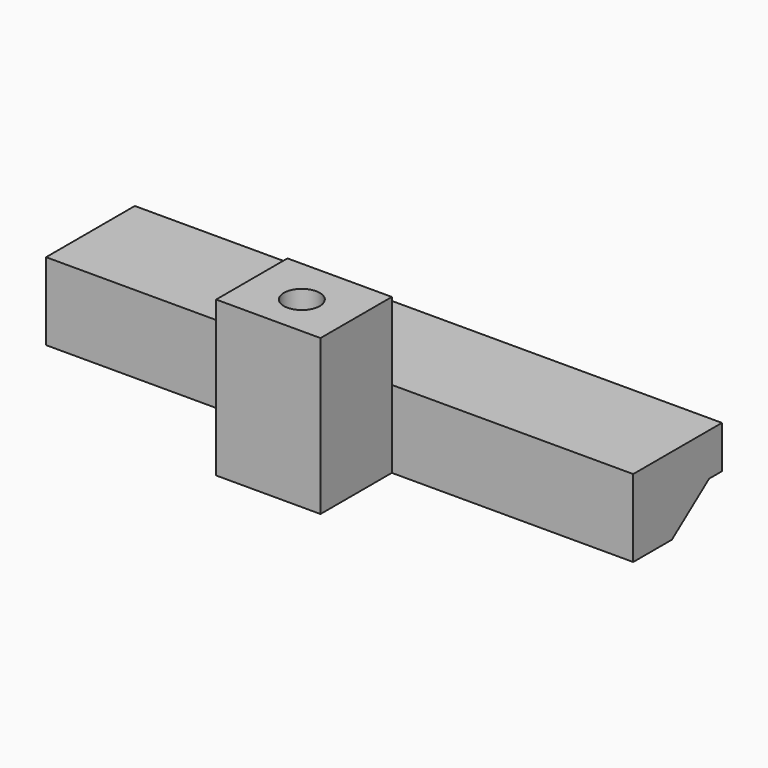
from build123d import *

# Parameters (mm, degrees)
F1_DEPTH    = 10.16
F0_W        = 13.6915519834
F0_H        = 11.6948671639
F2_DEPTH    = 20.32
F4_DEPTH    = 77.0159752498
F5_W        = 59.2985060066
F5_H        = 8.0565831158
F6_DEPTH    = 4.5666936785
F7_T1_DEPTH = 84.5685063134
F8_R        = 2.3549546022
F9_DEPTH    = 20.321


# Not quite as in the source:
# - a fillet or chamfer that OpenCascade refuses, or shapes differently, is made with other operations: its cross-section is extruded or revolved along the edge and cut away or added


with BuildPart() as f1:
    # F0 (on Top) → F1 (new body)
    with BuildSketch(Plane.XY):
        Polygon((38.5074876249, -7.2736367583), (38.5074876249, 7.2736367583), (-38.5074876249, 7.2736367583), (-38.5074876249, -7.2736367583), (-6.8457759917, -7.2736367583), (6.8457759917, -7.2736367583), align=None)
    extrude(amount=F1_DEPTH)

    # F0 (on Top) → F2 (join)
    with BuildSketch(Plane.XY):
        with Locations((0, -13.1210703403)):
            Rectangle(F0_W, F0_H)
    extrude(amount=F2_DEPTH)

    # F3 (on face) → F4 (cut, through all)
    with BuildSketch(Plane.YZ.offset(38.5074876249)):
        Polygon((5.1769153215, 4.5666936785), (1.6501703067, 1.9309354248), (-0.9334948961, 0), (7.2736367583, 0), (7.2736367583, 4.5666936785), align=None)
    extrude(amount=-F4_DEPTH, mode=Mode.SUBTRACT)

    # F5 (on face) → F6 (join, through all)
    with BuildSketch(Plane(origin=(0, 0, 4.5666936785), x_dir=(1, 0, 0), z_dir=(0, 0, -1))):
        with Locations((0.0417931005, -1.1486237636)):
            Rectangle(F5_W, F5_H)
    extrude(amount=F6_DEPTH)

    # F7: fillet of radius 5.08 on 1 edges, made by hand

    # F7_s2 → F7_t1 (cut)
    with BuildSketch(Plane.YZ.offset(-42.2424600562)):
        with BuildLine():
            ThreePointArc((0.1229152601, 0), (3.5287047345, 1.3107828324), (5.1769153215, 4.5666936785))
            Line((5.1769153215, 4.5666936785), (5.1769153215, 0))
            Line((5.1769153215, 0), (0.1229152601, 0))
        make_face()
    extrude(amount=F7_T1_DEPTH, mode=Mode.SUBTRACT)

    # F8 (on face) → F9 (cut, through all)
    with BuildSketch(Plane.XY.offset(20.32)):
        with Locations((0, -13.4750818834)):
            Circle(F8_R)
    extrude(amount=-F9_DEPTH, mode=Mode.SUBTRACT)


solid = f1.part
